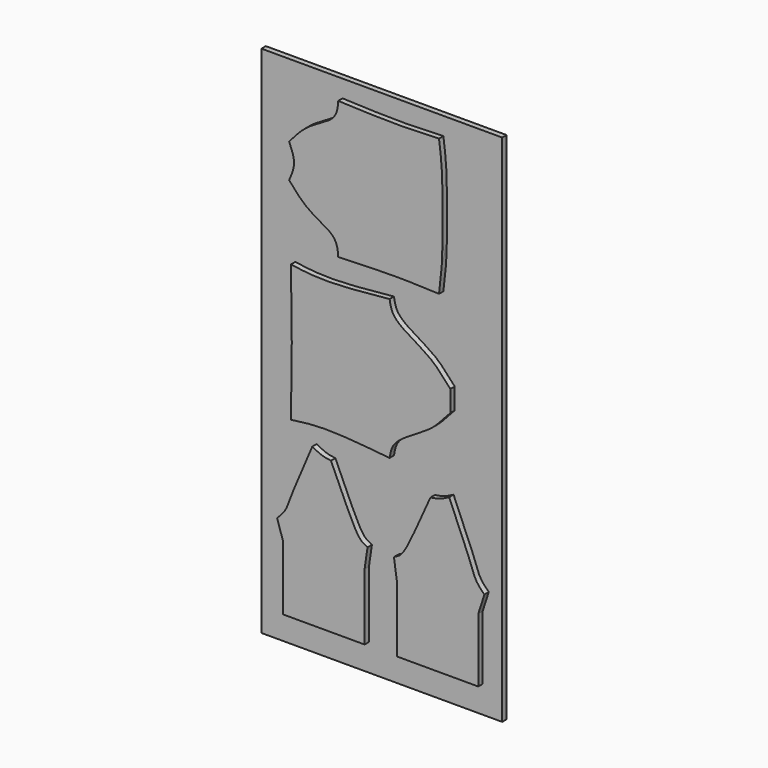
from build123d import *

# Parameters (mm, degrees)
F2_DEPTH = 25.4
F3_W     = 1117.6
F3_H     = 2387.6
F4_DEPTH = 25.4


# Not quite as in the source:
# - the dataset's text gives a spline's control points without its knots; the knots are read off the source's solid


with BuildPart() as f2:
    # F0 (on Front) → F2 (new body)
    with BuildSketch(Plane.XZ):
        with BuildLine():
            add(Edge.make_bspline(
                [(-19.3661805242, -304.1977286339), (-80.8509153389, -301.3951576074), (-215.7568387903, -295.2459331942), (-391.7817809144, -302.2462373132), (-487.5815808773, -306.0560822487)],
                knots=[0, 0, 0, 0, 0.4557600826, 1, 1, 1, 1], degree=3))
            add(Edge.make_bspline(
                [(-19.3661805242, -304.1977286339), (-12.0053351624, -250.6496178417), (-1.2323408104, -144.2686003565), (-2.9034086037, -39.0068169321), (-2.9034086037, 13.0084119737)],
                knots=[0, 0, 0, 0, 0.5032901479, 1, 1, 1, 1], degree=3))
            add(Edge.make_bspline(
                [(-19.3661805242, 330.2145525813), (-12.0053351624, 276.6664417891), (-1.2323408104, 170.2854243039), (-2.9034086037, 65.0236408795), (-2.9034086037, 13.0084119737)],
                knots=[0, 0, 0, 0, 0.5032901479, 1, 1, 1, 1], degree=3))
            add(Edge.make_bspline(
                [(-19.3661805242, 330.2145525813), (-80.8509153389, 327.4119815549), (-215.7568387903, 321.2627571417), (-391.7817809144, 328.2630612606), (-487.5815808773, 332.0729061961)],
                knots=[0, 0, 0, 0, 0.4557600826, 1, 1, 1, 1], degree=3))
            add(Edge.make_bspline(
                [(-714.9790525436, 91.8091461062), (-688.1054453065, 123.0561909313), (-635.963798658, 184.8539191183), (-525.8677553528, 234.0123661327), (-492.4773215799, 277.6462444761), (-488.000998717, 312.6780187869), (-487.5815808773, 332.0729061961)],
                knots=[0, 0, 0, 0, 0.3067591927, 0.6039732165, 0.7995556084, 1, 1, 1, 1], degree=3))
            add(Edge.make_bspline(
                [(-714.9790525436, 91.8091461062), (-703.6292552948, 65.5422347287), (-680.9296607971, 13.0084119737), (-703.6292552948, -39.5254107813), (-714.9790525436, -65.7923221588)],
                knots=[0, 0, 0, 0, 0.5, 1, 1, 1, 1], degree=3))
            add(Edge.make_bspline(
                [(-714.9790525436, -65.7923221588), (-688.1054453065, -97.0393669839), (-635.963798658, -158.8370951708), (-525.8677553528, -207.9955421852), (-492.4773215799, -251.6294205287), (-488.000998717, -286.6611948395), (-487.5815808773, -306.0560822487)],
                knots=[0, 0, 0, 0, 0.3067591927, 0.6039732165, 0.7995556084, 1, 1, 1, 1], degree=3))
        make_face()
    extrude(amount=F2_DEPTH)


with BuildPart() as f2b:
    # F1 (on Front) → F2, piece 2 (new body)
    with BuildSketch(Plane.XZ):
        with BuildLine():
            add(Edge.make_bspline(
                [(-228.6487041344, -1447.4794787136), (-218.9537680176, -1442.8331811079), (-196.0160951189, -1431.8403026208), (-159.0436729676, -1374.2670672458), (-99.2062321703, -1239.5307850908), (-58.9978663553, -1148.9933949677)],
                knots=[0, 0, 0, 0, 0.1936500421, 0.4581650944, 1, 1, 1, 1], degree=3))
            add(Edge.make_bspline(
                [(-214.9400903215, -1541.0479658065), (-219.5096282591, -1509.8584701089), (-224.0791661967, -1478.6689744113), (-228.6487041344, -1447.4794787136)],
                knots=[0, 0, 0, 0, 1, 1, 1, 1], degree=3))
            Line((-214.9400903215, -1541.0479658065), (-214.9400903215, -1849.3550693843))
            Line((-214.9400903215, -1849.3550693843), (162.8563435446, -1849.3550693843))
            Line((162.8563435446, -1849.3550693843), (162.8563435446, -1552.1766614882))
            add(Edge.make_bspline(
                [(191.2083061109, -1464.2927941648), (181.7576519221, -1493.5874166059), (172.3069977334, -1522.8820390471), (162.8563435446, -1552.1766614882)],
                knots=[0, 0, 0, 0, 1, 1, 1, 1], degree=3))
            add(Edge.make_bspline(
                [(27.8300525318, -1119.5806485382), (58.7260295475, -1191.1417299957), (106.9032959188, -1302.7296328945), (129.4230449419, -1363.6756023524), (150.6947810894, -1424.5121938967), (177.8604290666, -1451.1863917758), (191.2083061109, -1464.2927941648)],
                knots=[0, 0, 0, 0, 0.3803399346, 0.5930784559, 0.8000585614, 1, 1, 1, 1], degree=3))
            add(Edge.make_bspline(
                [(-58.9978663553, -1148.9933949677), (-45.7725702422, -1147.2922309278), (-17.6835949522, -1143.679158353), (12.0801469027, -1127.9198891038), (27.8300525318, -1119.5806485382)],
                knots=[0, 0, 0, 0, 0.4708358342, 1, 1, 1, 1], degree=3))
        make_face()
    extrude(amount=F2_DEPTH)


with BuildPart() as f2c:
    # F1 (on Front) → F2, piece 3 (new body)
    with BuildSketch(Plane.XZ):
        with BuildLine():
            Line((-364.8419774692, -1849.3550693843), (-364.8419774692, -1541.0479658065))
            add(Edge.make_bspline(
                [(-364.8419774692, -1541.0479658065), (-360.2724395316, -1509.8584701089), (-355.7029015939, -1478.6689744113), (-351.1333636563, -1447.4794787136)],
                knots=[0, 0, 0, 0, 1, 1, 1, 1], degree=3))
            add(Edge.make_bspline(
                [(-351.1333636563, -1447.4794787136), (-360.8282997731, -1442.8331811079), (-383.7659726718, -1431.8403026208), (-420.7383948231, -1374.2670672458), (-480.5758356204, -1239.5307850908), (-520.7842014354, -1148.9933949677)],
                knots=[0, 0, 0, 0, 0.1936500421, 0.4581650944, 1, 1, 1, 1], degree=3))
            add(Edge.make_bspline(
                [(-520.7842014354, -1148.9933949677), (-534.0094975485, -1147.2922309278), (-562.0984728385, -1143.679158353), (-591.8622146934, -1127.9198891038), (-607.6121203225, -1119.5806485382)],
                knots=[0, 0, 0, 0, 0.4708358342, 1, 1, 1, 1], degree=3))
            add(Edge.make_bspline(
                [(-607.6121203225, -1119.5806485382), (-638.5080973382, -1191.1417299957), (-686.6853637095, -1302.7296328945), (-709.2051127326, -1363.6756023524), (-730.4768488801, -1424.5121938967), (-757.6424968573, -1451.1863917758), (-770.9903739016, -1464.2927941648)],
                knots=[0, 0, 0, 0, 0.3803399346, 0.5930784559, 0.8000585614, 1, 1, 1, 1], degree=3))
            add(Edge.make_bspline(
                [(-770.9903739016, -1464.2927941648), (-761.5397197128, -1493.5874166059), (-752.089065524, -1522.8820390471), (-742.6384113353, -1552.1766614882)],
                knots=[0, 0, 0, 0, 1, 1, 1, 1], degree=3))
            Line((-742.6384113353, -1552.1766614882), (-742.6384113353, -1849.3550693843))
            Line((-742.6384113353, -1849.3550693843), (-364.8419774692, -1849.3550693843))
        make_face()
    extrude(amount=F2_DEPTH)


with BuildPart() as f2d:
    # F1 (on Front) → F2, piece 4 (new body)
    with BuildSketch(Plane.XZ):
        with BuildLine():
            add(Edge.make_bspline(
                [(-19.3661805242, 330.2145525813), (-80.8509153389, 327.4119815549), (-215.7568387903, 321.2627571417), (-391.7817809144, 328.2630612606), (-487.5815808773, 332.0729061961)],
                knots=[0, 0, 0, 0, 0.4557600826, 1, 1, 1, 1], degree=3))
            add(Edge.make_bspline(
                [(-487.5815808773, 332.0729061961), (-488.000998717, 312.6780187869), (-492.4773215799, 277.6462444761), (-525.8677553528, 234.0123661327), (-635.963798658, 184.8539191183), (-688.1054453065, 123.0561909313), (-714.9790525436, 91.8091461062)],
                knots=[0, 0, 0, 0, 0.2004443916, 0.3960267835, 0.6932408073, 1, 1, 1, 1], degree=3))
            add(Edge.make_bspline(
                [(-714.9790525436, 91.8091461062), (-703.6292552948, 65.5422347287), (-680.9296607971, 13.0084119737), (-703.6292552948, -39.5254107813), (-714.9790525436, -65.7923221588)],
                knots=[0, 0, 0, 0, 0.5, 1, 1, 1, 1], degree=3))
            add(Edge.make_bspline(
                [(-714.9790525436, -65.7923221588), (-688.1054453065, -97.0393669839), (-635.963798658, -158.8370951708), (-525.8677553528, -207.9955421852), (-492.4773215799, -251.6294205287), (-488.000998717, -286.6611948395), (-487.5815808773, -306.0560822487)],
                knots=[0, 0, 0, 0, 0.3067591927, 0.6039732165, 0.7995556084, 1, 1, 1, 1], degree=3))
            add(Edge.make_bspline(
                [(-487.5815808773, -306.0560822487), (-391.7817809144, -302.2462373132), (-215.7568387903, -295.2459331942), (-80.8509153389, -301.3951576074), (-19.3661805242, -304.1977286339)],
                knots=[0, 0, 0, 0, 0.5442399174, 1, 1, 1, 1], degree=3))
            add(Edge.make_bspline(
                [(-19.3661805242, -304.1977286339), (-12.0053351624, -250.6496178417), (-1.2323408104, -144.2686003565), (-2.9034086037, -39.0068169321), (-2.9034086037, 13.0084119737)],
                knots=[0, 0, 0, 0, 0.5032901479, 1, 1, 1, 1], degree=3))
            add(Edge.make_bspline(
                [(-2.9034086037, 13.0084119737), (-2.9034086037, 65.0236408795), (-1.2323408104, 170.2854243039), (-12.0053351624, 276.6664417891), (-19.3661805242, 330.2145525813)],
                knots=[0, 0, 0, 0, 0.4967098521, 1, 1, 1, 1], degree=3))
        make_face()
    extrude(amount=F2_DEPTH)


with BuildPart() as f2e:
    # F1 (on Front) → F2, piece 5 (new body)
    with BuildSketch(Plane.XZ):
        with BuildLine():
            add(Edge.make_bspline(
                [(33.1680851389, -773.8157648911), (33.1680851389, -738.939027458), (33.1680851389, -710.6132623747), (33.1680851389, -675.7365249416)],
                knots=[0, 0, 0, 0, 1, 1, 1, 1], degree=3))
            add(Edge.make_bspline(
                [(33.1680851389, -675.7365249416), (20.6098061512, -662.8767934516), (-4.3813482561, -634.8395333098), (-51.3009460882, -582.2261877467), (-139.4460358283, -530.7951922079), (-200.8186488979, -492.0300492954), (-239.2845563093, -453.2698961725), (-245.6035321453, -417.9393915327), (-248.7929982733, -400.0977984016)],
                knots=[0, 0, 0, 0, 0.1506791965, 0.322350645, 0.5298093251, 0.7055655926, 0.8516945833, 1, 1, 1, 1], degree=3))
            add(Edge.make_bspline(
                [(-248.7929982733, -400.0977984016), (-322.8442956619, -407.4236513718), (-456.7914302975, -420.6749656462), (-597.7353998354, -422.6870039331), (-671.8963425102, -412.2940111542), (-706.5266592097, -407.4408820217)],
                knots=[0, 0, 0, 0, 0.3972322443, 0.7185305698, 1, 1, 1, 1], degree=3))
            add(Edge.make_bspline(
                [(-706.5266592097, -407.4408820217), (-705.2643719108, -513.2193029866), (-704.002084612, -618.9977239515), (-702.7397973131, -724.7761449163)],
                knots=[0, 0, 0, 0, 1, 1, 1, 1], degree=3))
            add(Edge.make_bspline(
                [(-702.7397973131, -724.7761449163), (-704.002084612, -830.5545658812), (-705.2643719108, -936.3329868461), (-706.5266592097, -1042.111407811)],
                knots=[0, 0, 0, 0, 1, 1, 1, 1], degree=3))
            add(Edge.make_bspline(
                [(-706.5266592097, -1042.111407811), (-671.8963425102, -1037.2582786785), (-597.7353998354, -1026.8652858996), (-456.7914302975, -1028.8773241865), (-322.8442956619, -1042.1286384609), (-248.7929982733, -1049.4544914311)],
                knots=[0, 0, 0, 0, 0.2814694302, 0.6027677557, 1, 1, 1, 1], degree=3))
            add(Edge.make_bspline(
                [(-248.7929982733, -1049.4544914311), (-245.6035321453, -1031.6128982999), (-239.2845563093, -996.2823936602), (-200.8186488979, -957.5222405373), (-139.4460358283, -918.7570976248), (-51.3009460882, -867.326102086), (-4.3813482561, -814.7127565229), (20.6098061512, -786.6754963811), (33.1680851389, -773.8157648911)],
                knots=[0, 0, 0, 0, 0.1483054167, 0.2944344074, 0.4701906749, 0.677649355, 0.8493208035, 1, 1, 1, 1], degree=3))
        make_face()
    extrude(amount=F2_DEPTH)


with BuildPart() as f4:
    # F3 (on face) → F4 (new body)
    with BuildSketch(Plane(origin=(0, 0, 0), x_dir=(-1, 0, 0), z_dir=(0, 1, 0))):
        with Locations((305.172461319, -781.0237682343)):
            Rectangle(F3_W, F3_H)
        with BuildLine():
            add(Edge.make_bspline(
                [(19.3661805242, -304.1977286339), (12.0053351624, -250.6496178417), (1.2323408104, -144.2686003565), (2.9034086037, -39.0068169321), (2.9034086037, 13.0084119737)],
                knots=[0, 0, 0, 0, 0.5032901479, 1, 1, 1, 1], degree=3))
            add(Edge.make_bspline(
                [(2.9034086037, 13.0084119737), (2.9034086037, 65.0236408795), (1.2323408104, 170.2854243039), (12.0053351624, 276.6664417891), (19.3661805242, 330.2145525813)],
                knots=[0, 0, 0, 0, 0.4967098521, 1, 1, 1, 1], degree=3))
            add(Edge.make_bspline(
                [(19.3661805242, 330.2145525813), (80.8509153389, 327.4119815549), (215.7568387903, 321.2627571417), (391.7817809144, 328.2630612606), (487.5815808773, 332.0729061961)],
                knots=[0, 0, 0, 0, 0.4557600826, 1, 1, 1, 1], degree=3))
            add(Edge.make_bspline(
                [(487.5815808773, 332.0729061961), (488.000998717, 312.6780187869), (492.4773215799, 277.6462444761), (525.8677553528, 234.0123661327), (635.963798658, 184.8539191183), (688.1054453065, 123.0561909313), (714.9790525436, 91.8091461062)],
                knots=[0, 0, 0, 0, 0.2004443916, 0.3960267835, 0.6932408073, 1, 1, 1, 1], degree=3))
            add(Edge.make_bspline(
                [(714.9790525436, 91.8091461062), (703.6292552948, 65.5422347287), (680.9296607971, 13.0084119737), (703.6292552948, -39.5254107813), (714.9790525436, -65.7923221588)],
                knots=[0, 0, 0, 0, 0.5, 1, 1, 1, 1], degree=3))
            add(Edge.make_bspline(
                [(714.9790525436, -65.7923221588), (688.1054453065, -97.0393669839), (635.963798658, -158.8370951708), (525.8677553528, -207.9955421852), (492.4773215799, -251.6294205287), (488.000998717, -286.6611948395), (487.5815808773, -306.0560822487)],
                knots=[0, 0, 0, 0, 0.3067591927, 0.6039732165, 0.7995556084, 1, 1, 1, 1], degree=3))
            add(Edge.make_bspline(
                [(487.5815808773, -306.0560822487), (391.7817809144, -302.2462373132), (215.7568387903, -295.2459331942), (80.8509153389, -301.3951576074), (19.3661805242, -304.1977286339)],
                knots=[0, 0, 0, 0, 0.5442399174, 1, 1, 1, 1], degree=3))
        make_face(mode=Mode.SUBTRACT)
        with BuildLine():
            add(Edge.make_bspline(
                [(2.9034086037, 13.0084119737), (2.9034086037, 65.0236408795), (1.2323408104, 170.2854243039), (12.0053351624, 276.6664417891), (19.3661805242, 330.2145525813)],
                knots=[0, 0, 0, 0, 0.4967098521, 1, 1, 1, 1], degree=3))
            add(Edge.make_bspline(
                [(19.3661805242, -304.1977286339), (12.0053351624, -250.6496178417), (1.2323408104, -144.2686003565), (2.9034086037, -39.0068169321), (2.9034086037, 13.0084119737)],
                knots=[0, 0, 0, 0, 0.5032901479, 1, 1, 1, 1], degree=3))
            add(Edge.make_bspline(
                [(487.5815808773, -306.0560822487), (391.7817809144, -302.2462373132), (215.7568387903, -295.2459331942), (80.8509153389, -301.3951576074), (19.3661805242, -304.1977286339)],
                knots=[0, 0, 0, 0, 0.5442399174, 1, 1, 1, 1], degree=3))
            add(Edge.make_bspline(
                [(714.9790525436, -65.7923221588), (688.1054453065, -97.0393669839), (635.963798658, -158.8370951708), (525.8677553528, -207.9955421852), (492.4773215799, -251.6294205287), (488.000998717, -286.6611948395), (487.5815808773, -306.0560822487)],
                knots=[0, 0, 0, 0, 0.3067591927, 0.6039732165, 0.7995556084, 1, 1, 1, 1], degree=3))
            add(Edge.make_bspline(
                [(714.9790525436, 91.8091461062), (703.6292552948, 65.5422347287), (680.9296607971, 13.0084119737), (703.6292552948, -39.5254107813), (714.9790525436, -65.7923221588)],
                knots=[0, 0, 0, 0, 0.5, 1, 1, 1, 1], degree=3))
            add(Edge.make_bspline(
                [(487.5815808773, 332.0729061961), (488.000998717, 312.6780187869), (492.4773215799, 277.6462444761), (525.8677553528, 234.0123661327), (635.963798658, 184.8539191183), (688.1054453065, 123.0561909313), (714.9790525436, 91.8091461062)],
                knots=[0, 0, 0, 0, 0.2004443916, 0.3960267835, 0.6932408073, 1, 1, 1, 1], degree=3))
            add(Edge.make_bspline(
                [(19.3661805242, 330.2145525813), (80.8509153389, 327.4119815549), (215.7568387903, 321.2627571417), (391.7817809144, 328.2630612606), (487.5815808773, 332.0729061961)],
                knots=[0, 0, 0, 0, 0.4557600826, 1, 1, 1, 1], degree=3))
        make_face()
    extrude(amount=F4_DEPTH)


solid = Compound([f2.part, f2b.part, f2c.part, f2d.part, f2e.part, f4.part])
